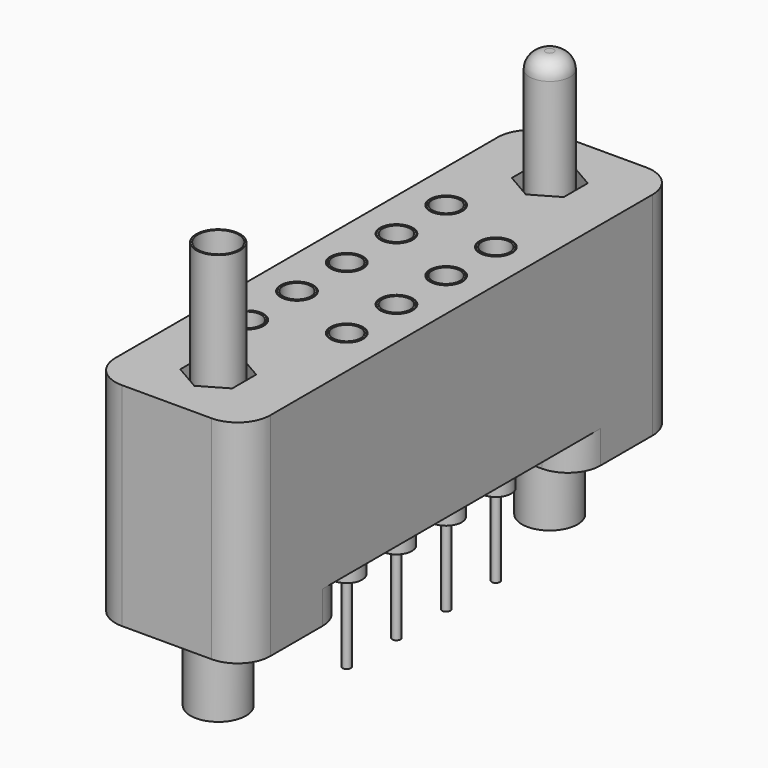
from build123d import *

# Parameters (mm, degrees)
F0_W      = 9.5
F0_H      = 33.3
F0_R      = 1
F1_DEPTH  = 13
F2_W      = 17.3
F2_H      = 4
F3_DEPTH  = 9.501
F4_R      = 2
F5_R      = 0.25
F6_DEPTH  = 5
F7_R      = 0.95
F8_DEPTH  = 13
F9_T      = -0.1
F9_2_T    = -0.1
F9_3_T    = -0.1
F9_4_T    = -0.1
F9_5_T    = -0.1
F9_6_T    = -0.1
F9_7_T    = -0.1
F9_8_T    = -0.1
F9_9_T    = -0.1
F10_R     = 1.25
F11_DEPTH = 20
F10_R_2   = 1.35
F12_R     = 1
F13_R     = 1.7
F14_DEPTH = 5
F15_T     = -0.1


# Not quite as in the source:
# - a feature names something its author has since deleted; it is built from what else it names


with BuildPart() as f1:
    # F0 (on Top) → F1 (new body)
    with BuildSketch(Plane.XY):
        Rectangle(F0_W, F0_H)
        with Locations((-2.285, -7.62)):
            Circle(F0_R, mode=Mode.SUBTRACT)
        with Locations((-2.285, -3.81)):
            Circle(F0_R, mode=Mode.SUBTRACT)
        Polygon((0, -14.5374084972), (-1.5912424357, -13.6187042486), (-1.5912424357, -11.7812957514), (0, -10.8625915028), (1.5912424357, -11.7812957514), (1.5912424357, -13.6187042486), align=None, mode=Mode.SUBTRACT)
        with Locations((2.285, -5.715)):
            Circle(F0_R, mode=Mode.SUBTRACT)
        with Locations((2.285, -1.905)):
            Circle(F0_R, mode=Mode.SUBTRACT)
        with Locations((-2.285, 0)):
            Circle(F0_R, mode=Mode.SUBTRACT)
        with Locations((-2.285, 3.81)):
            Circle(F0_R, mode=Mode.SUBTRACT)
        with Locations((-2.285, 7.62)):
            Circle(F0_R, mode=Mode.SUBTRACT)
        with Locations((2.285, 1.905)):
            Circle(F0_R, mode=Mode.SUBTRACT)
        with Locations((2.285, 5.715)):
            Circle(F0_R, mode=Mode.SUBTRACT)
        Polygon((0, 14.5374084972), (1.5912424357, 13.6187042486), (1.5912424357, 11.7812957514), (0, 10.8625915028), (-1.5912424357, 11.7812957514), (-1.5912424357, 13.6187042486), align=None, mode=Mode.SUBTRACT)
    extrude(amount=F1_DEPTH)

    # F2 (on face) → F3 (cut, through all)
    with BuildSketch(Plane.YZ.offset(4.75)):
        Rectangle(F2_W, F2_H)
    extrude(amount=-F3_DEPTH, mode=Mode.SUBTRACT)

    # F4
    f4_edges = [f1.edges().sort_by_distance(p)[0] for p in [
        (4.75, -16.65, 6.5),
        (-4.75, -16.65, 6.5),
        (4.75, 16.65, 6.5),
        (-4.75, 16.65, 6.5),
        (-4.75, -8.65, 1),
        (-4.75, 8.65, 1),
        (4.75, 8.65, 1),
        (4.75, -8.65, 1),
    ]]
    fillet(f4_edges, radius=F4_R)


with BuildPart() as f6:
    # F5 (on face) → F6 (new body)
    with BuildSketch(Plane.XY):
        with Locations((-2.285, 7.62)):
            Circle(F5_R)
    extrude(amount=-F6_DEPTH)

    # F7 (on face) → F8 (join)
    with BuildSketch(Plane.XY):
        with Locations((-2.285, 7.62)):
            Circle(F7_R)
    extrude(amount=F8_DEPTH)

    # F9
    f9_openings = [f6.faces().sort_by_distance(p)[0] for p in [
        (-2.285, 7.62, 13),
    ]]
    offset(amount=F9_T, openings=f9_openings, kind=Kind.INTERSECTION)


with BuildPart() as f6b:
    # F5 (on face) → F6, piece 2 (new body)
    with BuildSketch(Plane.XY):
        with Locations((-2.285, 3.81)):
            Circle(F5_R)
    extrude(amount=-F6_DEPTH)


with BuildPart() as f6c:
    # F5 (on face) → F6, piece 3 (new body)
    with BuildSketch(Plane.XY):
        with Locations((2.285, 1.905)):
            Circle(F5_R)
    extrude(amount=-F6_DEPTH)


with BuildPart() as f6d:
    # F5 (on face) → F6, piece 4 (new body)
    with BuildSketch(Plane.XY):
        with Locations((2.285, 5.715)):
            Circle(F5_R)
    extrude(amount=-F6_DEPTH)


with BuildPart() as f6e:
    # F5 (on face) → F6, piece 5 (new body)
    with BuildSketch(Plane.XY):
        with Locations((-2.285, 0)):
            Circle(F5_R)
    extrude(amount=-F6_DEPTH)


with BuildPart() as f6f:
    # F5 (on face) → F6, piece 6 (new body)
    with BuildSketch(Plane.XY):
        with Locations((-2.285, -3.81)):
            Circle(F5_R)
    extrude(amount=-F6_DEPTH)


with BuildPart() as f6g:
    # F5 (on face) → F6, piece 7 (new body)
    with BuildSketch(Plane.XY):
        with Locations((-2.285, -7.62)):
            Circle(F5_R)
    extrude(amount=-F6_DEPTH)


with BuildPart() as f6h:
    # F5 (on face) → F6, piece 8 (new body)
    with BuildSketch(Plane.XY):
        with Locations((2.285, -5.715)):
            Circle(F5_R)
    extrude(amount=-F6_DEPTH)


with BuildPart() as f6i:
    # F5 (on face) → F6, piece 9 (new body)
    with BuildSketch(Plane.XY):
        with Locations((2.285, -1.905)):
            Circle(F5_R)
    extrude(amount=-F6_DEPTH)


with BuildPart() as f8:
    # F7 (on face) → F8, piece 2 (new body)
    with BuildSketch(Plane.XY):
        with Locations((-2.285, 3.81)):
            Circle(F7_R)
    extrude(amount=F8_DEPTH)

    # F9#3
    f9_3_openings = [f8.faces().sort_by_distance(p)[0] for p in [
        (-2.285, 3.81, 13),
    ]]
    offset(amount=F9_3_T, openings=f9_3_openings)


with BuildPart() as f8b:
    # F7 (on face) → F8, piece 3 (new body)
    with BuildSketch(Plane.XY):
        with Locations((2.285, 5.715)):
            Circle(F7_R)
    extrude(amount=F8_DEPTH)

    # F9#2
    f9_2_openings = [f8b.faces().sort_by_distance(p)[0] for p in [
        (2.285, 5.715, 13),
    ]]
    offset(amount=F9_2_T, openings=f9_2_openings)


with BuildPart() as f8c:
    # F7 (on face) → F8, piece 4 (new body)
    with BuildSketch(Plane.XY):
        with Locations((2.285, 1.905)):
            Circle(F7_R)
    extrude(amount=F8_DEPTH)

    # F9#4
    f9_4_openings = [f8c.faces().sort_by_distance(p)[0] for p in [
        (2.285, 1.905, 13),
    ]]
    offset(amount=F9_4_T, openings=f9_4_openings)


with BuildPart() as f8d:
    # F7 (on face) → F8, piece 5 (new body)
    with BuildSketch(Plane.XY):
        with Locations((-2.285, 0)):
            Circle(F7_R)
    extrude(amount=F8_DEPTH)

    # F9#5
    f9_5_openings = [f8d.faces().sort_by_distance(p)[0] for p in [
        (-2.285, 0, 13),
    ]]
    offset(amount=F9_5_T, openings=f9_5_openings)


with BuildPart() as f8e:
    # F7 (on face) → F8, piece 6 (new body)
    with BuildSketch(Plane.XY):
        with Locations((-2.285, -3.81)):
            Circle(F7_R)
    extrude(amount=F8_DEPTH)

    # F9#6
    f9_6_openings = [f8e.faces().sort_by_distance(p)[0] for p in [
        (-2.285, -3.81, 13),
    ]]
    offset(amount=F9_6_T, openings=f9_6_openings)


with BuildPart() as f8f:
    # F7 (on face) → F8, piece 7 (new body)
    with BuildSketch(Plane.XY):
        with Locations((-2.285, -7.62)):
            Circle(F7_R)
    extrude(amount=F8_DEPTH)

    # F9#9
    f9_9_openings = [f8f.faces().sort_by_distance(p)[0] for p in [
        (-2.285, -7.62, 13),
    ]]
    offset(amount=F9_9_T, openings=f9_9_openings)


with BuildPart() as f8g:
    # F7 (on face) → F8, piece 8 (new body)
    with BuildSketch(Plane.XY):
        with Locations((2.285, -1.905)):
            Circle(F7_R)
    extrude(amount=F8_DEPTH)

    # F9#7
    f9_7_openings = [f8g.faces().sort_by_distance(p)[0] for p in [
        (2.285, -1.905, 13),
    ]]
    offset(amount=F9_7_T, openings=f9_7_openings)


with BuildPart() as f8h:
    # F7 (on face) → F8, piece 9 (new body)
    with BuildSketch(Plane.XY):
        with Locations((2.285, -5.715)):
            Circle(F7_R)
    extrude(amount=F8_DEPTH)

    # F9#8
    f9_8_openings = [f8h.faces().sort_by_distance(p)[0] for p in [
        (2.285, -5.715, 13),
    ]]
    offset(amount=F9_8_T, openings=f9_8_openings)


with BuildPart() as f11:
    # F10 (on face) → F11 (new body)
    with BuildSketch(Plane.XY):
        with Locations((0, 12.7)):
            Circle(F10_R)
    extrude(amount=F11_DEPTH)

    # F12
    f12_edges = [f11.edges().sort_by_distance(p)[0] for p in [
        (-1.25, 12.7, 20),
    ]]
    fillet(f12_edges, radius=F12_R)


with BuildPart() as f11b:
    # F10 (on face) → F11, piece 2 (new body)
    with BuildSketch(Plane.XY):
        with Locations((0, -12.7)):
            Circle(F10_R_2)
    extrude(amount=F11_DEPTH)

    # F15
    f15_openings = [f11b.faces().sort_by_distance(p)[0] for p in [
        (0, -12.7, 20),
    ]]
    offset(amount=F15_T, openings=f15_openings)


with BuildPart() as f14:
    # F13 (on face) → F14 (new body)
    with BuildSketch(Plane.XY):
        with Locations((0, 12.7)):
            Circle(F13_R)
    extrude(amount=-F14_DEPTH)


with BuildPart() as f14b:
    # F13 (on face) → F14, piece 2 (new body)
    with BuildSketch(Plane.XY):
        with Locations((0, -12.7)):
            Circle(F13_R)
    extrude(amount=-F14_DEPTH)


solid = Compound([f1.part, f6.part, f6b.part, f6c.part, f6d.part, f6e.part, f6f.part, f6g.part, f6h.part, f6i.part, f8.part, f8b.part, f8c.part, f8d.part, f8e.part, f8f.part, f8g.part, f8h.part, f11.part, f11b.part, f14.part, f14b.part])
